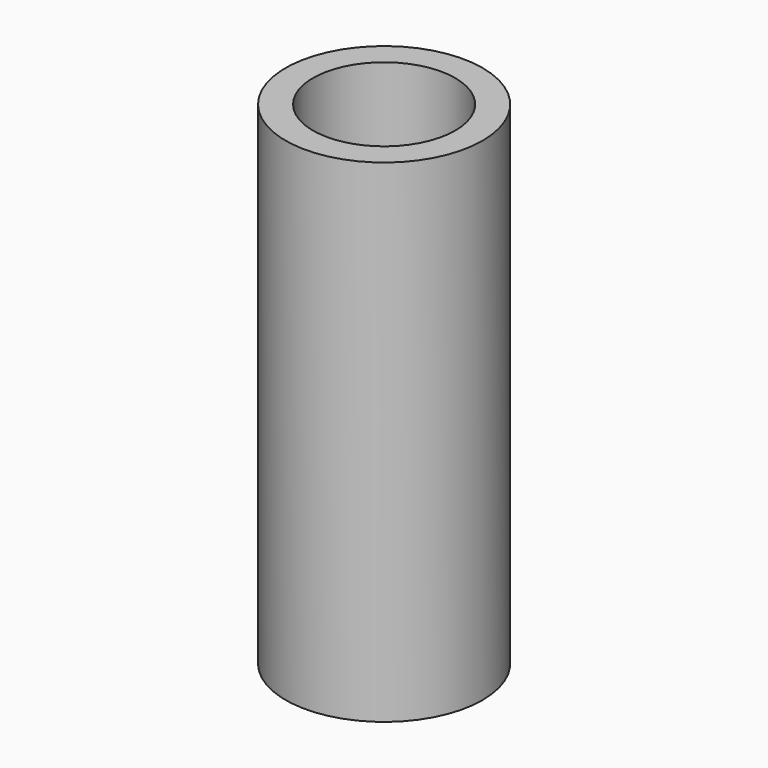
from build123d import *

# Parameters (mm, degrees)
F0_R     = 9
F0_R_2   = 6.5
F1_DEPTH = 45


# Not quite as in the source:
# - the program builds the solid bodies; features that only make, move or delete a surface that nothing else refers to are left out


with BuildPart() as f1:
    # F0 (on Top) → F1 (new body)
    with BuildSketch(Plane.XY):
        Circle(F0_R)
        Circle(F0_R_2, mode=Mode.SUBTRACT)
    extrude(amount=F1_DEPTH)


solid = f1.part
